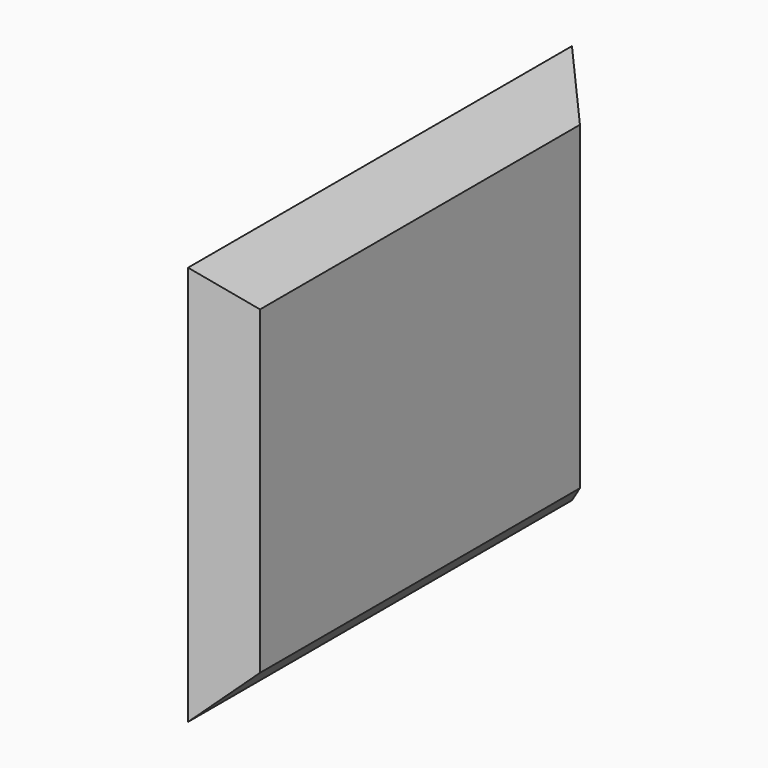
from build123d import *

# Parameters (mm, degrees)
F0_W     = 300
F0_H     = 250
F1_DEPTH = 25
F2_SIZE  = 24.99999


# Not quite as in the source:
# - a fillet or chamfer is up to 0.001 mm smaller than in the source, because OpenCascade refuses the exact size


with BuildPart() as f1:
    # F0 (on Right) → F1 (new body)
    with BuildSketch(Plane.YZ):
        Rectangle(F0_W, F0_H)
    extrude(amount=-F1_DEPTH)

    # F2 (size 25 in the source; OpenCascade refuses exactly that, so slightly less here)
    f2_edges = [f1.edges().sort_by_distance(p)[0] for p in [
        (0, 0, 125),
        (0, -150, 0),
        (0, 0, -125),
        (0, 150, 0),
    ]]
    chamfer(f2_edges, length=F2_SIZE)


solid = f1.part
